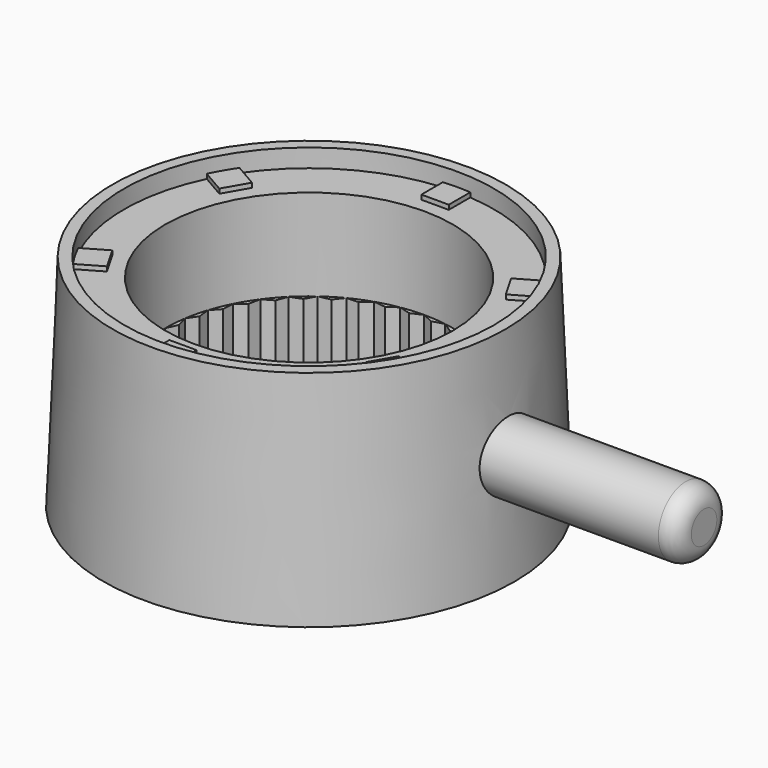
from build123d import *

# Parameters (mm, degrees)
F0_R           = 22.5
F2_R           = 21.5
F4_R           = 20.25
F5_DEPTH       = 2
F6_R           = 21.75
F7_DEPTH       = 3.5
F8_R           = 15.75
F9_DEPTH       = 18.5
F10_W          = 3
F10_H          = 3
F11_DEPTH      = 0.5
F14_R          = 16
F15_DEPTH      = 8.5
F15_DEPTH_BACK = 0.5
F18_R          = 3.75
F19_DEPTH      = 23
F20_R          = 2


with BuildPart() as f3:
    # F0 (on Top) → F3 section 0
    with BuildSketch(Plane.XY):
        Circle(F0_R)
    # F2 (on offset) → F3 section 1
    with BuildSketch(Plane.XY.offset(24)):
        Circle(F2_R)
    loft()

    # F4 (on face) → F5 (cut)
    with BuildSketch(Plane.XY.offset(24)):
        Circle(F4_R)
    extrude(amount=-F5_DEPTH, mode=Mode.SUBTRACT)

    # F6 (on face) → F7 (cut)
    with BuildSketch(Plane(origin=(0, 0, 0), x_dir=(1, 0, 0), z_dir=(0, 0, -1))):
        Circle(F6_R)
    extrude(amount=-F7_DEPTH, mode=Mode.SUBTRACT)

    # F8 (on face) → F9 (cut, through all)
    with BuildSketch(Plane.XY.offset(22)):
        Circle(F8_R)
    extrude(amount=-F9_DEPTH, mode=Mode.SUBTRACT)

    # F10 (on face) → F11 (join)
    with BuildSketch(Plane.XY.offset(22)):
        with Locations((0, 18.75)):
            Rectangle(F10_W, F10_H)
        Polygon((-15.6889382153, 7.3259618943), (-14.1889382153, 9.9240381057), (-16.7870144266, 11.4240381057), (-18.2870144266, 8.8259618943), align=None)
        Polygon((-14.1889382153, -9.9240381057), (-15.6889382153, -7.3259618943), (-18.2870144266, -8.8259618943), (-16.7870144266, -11.4240381057), align=None)
        with Locations((0, -18.75)):
            Rectangle(F10_W, F10_H)
        Polygon((15.6889382153, -7.3259618943), (14.1889382153, -9.9240381057), (16.7870144266, -11.4240381057), (18.2870144266, -8.8259618943), align=None)
        Polygon((14.1889382153, 9.9240381057), (15.6889382153, 7.3259618943), (18.2870144266, 8.8259618943), (16.7870144266, 11.4240381057), align=None)
    extrude(amount=F11_DEPTH)

    # F14 (on face) → F15 (join, two sides)
    with BuildSketch(Plane(origin=(0, 0, 3.5), x_dir=(1, 0, 0), z_dir=(0, 0, -1))) as f15_sk:
        Circle(F14_R)
        Polygon((-1.1965012098, 15.2029893394), (0, 15.75), (1.1965012098, 15.2029893394), (2.4638428244, 15.5560913644), (3.5600417988, 14.8286412861), (4.8670176614, 14.9791401316), (5.8359223436, 14.0891628708), (7.1503503709, 14.033352756), (7.9681031119, 13.0027625064), (9.2576177236, 12.7420176614), (9.904082737, 11.5961909754), (11.1369318037, 11.1369318037), (11.5961909754, 9.904082737), (12.7420176614, 9.2576177236), (13.0027625064, 7.9681031119), (14.033352756, 7.1503503709), (14.0891628708, 5.8359223436), (14.9791401316, 4.8670176614), (14.8286412861, 3.5600417988), (15.5560913644, 2.4638428244), (15.2029893394, 1.1965012098), (15.75, 0), (15.2029893394, -1.1965012098), (15.5560913644, -2.4638428244), (14.8286412861, -3.5600417988), (14.9791401316, -4.8670176614), (14.0891628708, -5.8359223436), (14.033352756, -7.1503503709), (13.0027625064, -7.9681031119), (12.7420176614, -9.2576177236), (11.5961909754, -9.904082737), (11.1369318037, -11.1369318037), (9.904082737, -11.5961909754), (9.2576177236, -12.7420176614), (7.9681031119, -13.0027625064), (7.1503503709, -14.033352756), (5.8359223436, -14.0891628708), (4.8670176614, -14.9791401316), (3.5600417988, -14.8286412861), (2.4638428244, -15.5560913644), (1.1965012098, -15.2029893394), (0, -15.75), (-1.1965012098, -15.2029893394), (-2.4638428244, -15.5560913644), (-3.5600417988, -14.8286412861), (-4.8670176614, -14.9791401316), (-5.8359223436, -14.0891628708), (-7.1503503709, -14.033352756), (-7.9681031119, -13.0027625064), (-9.2576177236, -12.7420176614), (-9.904082737, -11.5961909754), (-11.1369318037, -11.1369318037), (-11.5961909754, -9.904082737), (-12.7420176614, -9.2576177236), (-13.0027625064, -7.9681031119), (-14.033352756, -7.1503503709), (-14.0891628708, -5.8359223436), (-14.9791401316, -4.8670176614), (-14.8286412861, -3.5600417988), (-15.5560913644, -2.4638428244), (-15.2029893394, -1.1965012098), (-15.75, 0), (-15.2029893394, 1.1965012098), (-15.5560913644, 2.4638428244), (-14.8286412861, 3.5600417988), (-14.9791401316, 4.8670176614), (-14.0891628708, 5.8359223436), (-14.033352756, 7.1503503709), (-13.0027625064, 7.9681031119), (-12.7420176614, 9.2576177236), (-11.5961909754, 9.904082737), (-11.1369318037, 11.1369318037), (-9.904082737, 11.5961909754), (-9.2576177236, 12.7420176614), (-7.9681031119, 13.0027625064), (-7.1503503709, 14.033352756), (-5.8359223436, 14.0891628708), (-4.8670176614, 14.9791401316), (-3.5600417988, 14.8286412861), (-2.4638428244, 15.5560913644), align=None, mode=Mode.SUBTRACT)
    extrude(amount=-F15_DEPTH)
    extrude(f15_sk.sketch, amount=F15_DEPTH_BACK)

    # F18 (on offset) → F19 (join)
    with BuildSketch(Plane.YZ.offset(20.25)):
        with Locations((0, 12)):
            Circle(F18_R)
    extrude(amount=F19_DEPTH)

    # F20
    f20_edges = [f3.edges().sort_by_distance(p)[0] for p in [
        (43.25, -3.75, 12),
    ]]
    fillet(f20_edges, radius=F20_R)


solid = f3.part
